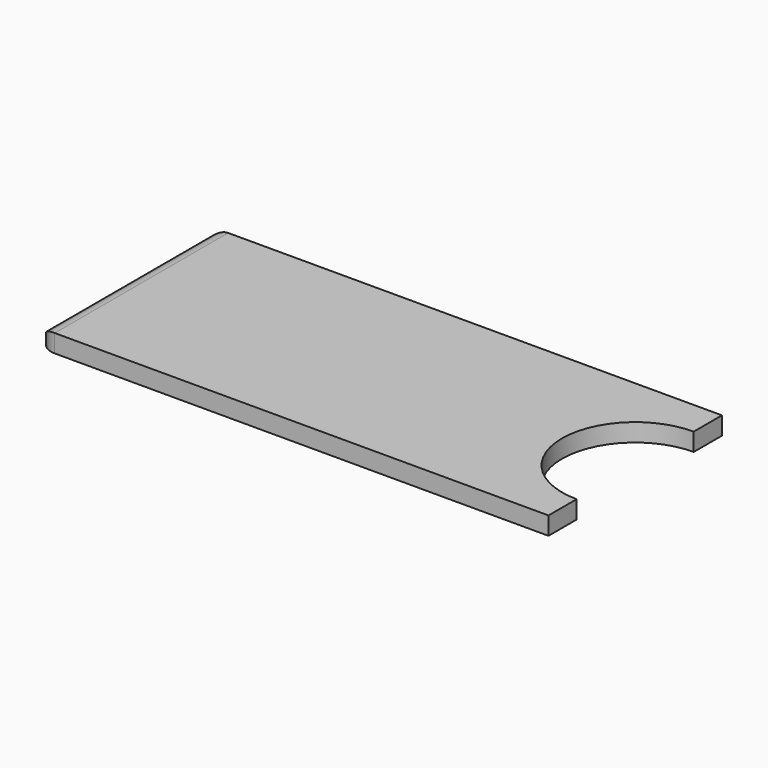
from build123d import *

# Parameters (mm, degrees)
F1_DEPTH = 2
F2_R     = 1.99999


# Not quite as in the source:
# - a fillet or chamfer is up to 0.001 mm smaller than in the source, because OpenCascade refuses the exact size


with BuildPart() as f1:
    # F0 (on Top) → F1 (new body)
    with BuildSketch(Plane.XY):
        with BuildLine():
            Line((-34.2, -12.075), (22.8, -12.075))
            Line((22.8, -12.075), (22.8, -8.15))
            ThreePointArc((22.8, -8.15), (14.65, 0), (22.8, 8.15))
            Line((22.8, 8.15), (22.8, 12.075))
            Line((22.8, 12.075), (-34.2, 12.075))
            Line((-34.2, 12.075), (-34.2, -12.075))
        make_face()
    extrude(amount=F1_DEPTH)

    # F2 (radius 2 in the source; OpenCascade refuses exactly that, so slightly less here)
    f2_edges = [f1.edges().sort_by_distance(p)[0] for p in [
        (-34.2, -12.075, 1),
        (-34.2, 12.075, 1),
        (-34.2, 0, 2),
    ]]
    fillet(f2_edges, radius=F2_R)


solid = f1.part
